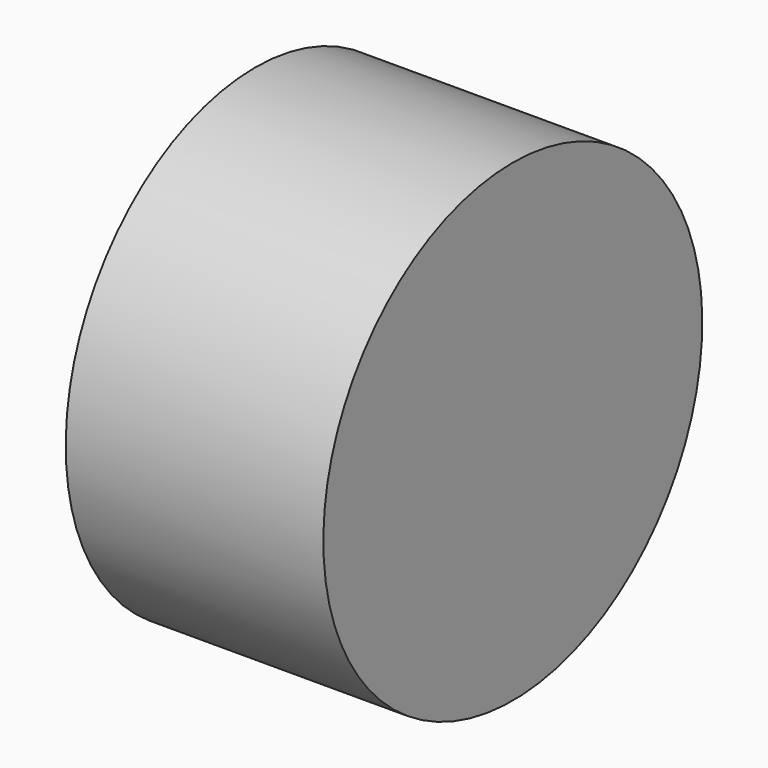
from build123d import *

# Parameters (mm, degrees)
F0_W = 45.8932034671
F0_H = 42.1916022897


# Not quite as in the source:
# - the program builds the solid bodies; features that only make, move or delete a surface that nothing else refers to are left out


with BuildPart() as f1:
    # F0 (on Front) → F1 (revolve)
    with BuildSketch(Plane.XZ):
        with Locations((22.9466017336, 21.0958011448)):
            Rectangle(F0_W, F0_H)
    revolve(axis=Axis((22.9466017336, 0, 0), (1, 0, 0)))


solid = f1.part
